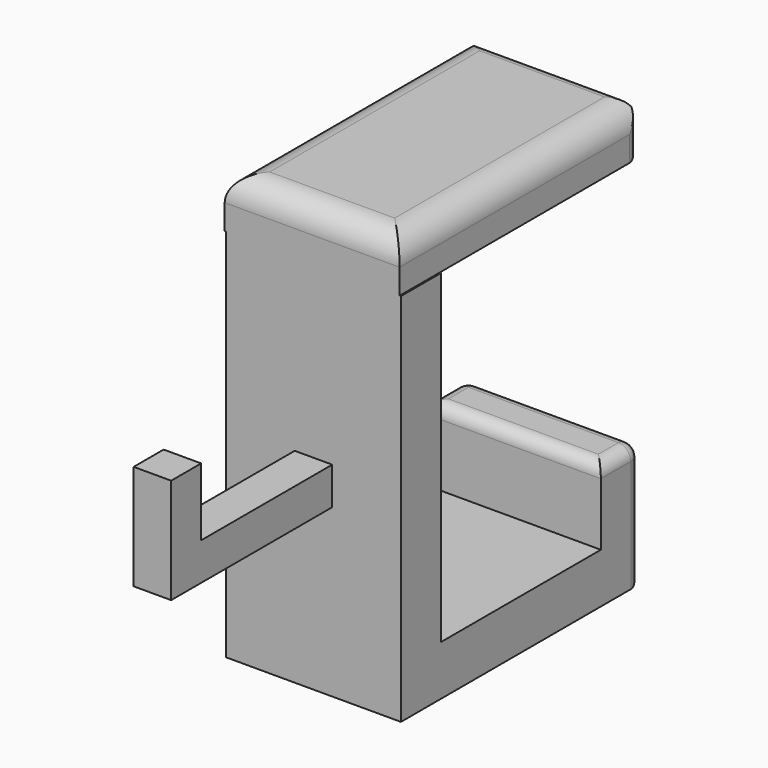
from build123d import *

# Parameters (mm, degrees)
F1_W         = 17.78
F1_H         = 30.48
F2_DEPTH     = 5.08
F3_W         = 17.78
F3_H         = 5.08
F4_DEPTH     = 38.1
F6_W         = 17.78
F6_H         = 5.08
F7_DEPTH     = 25.4
F9_W         = 17.78
F9_H         = 5.08
F10_DEPTH    = 7.62
F11_R        = 1.27
F12_R        = 1.27
F13_T1_DEPTH = 41.91
F13_T3_DEPTH = 30.48
F16_DEPTH    = 1.905


# Not quite as in the source:
# - a fillet or chamfer that OpenCascade refuses, or shapes differently, is made with other operations: its cross-section is extruded or revolved along the edge and cut away or added


with BuildPart() as f2:
    # F1 (on offset) → F2 (new body)
    with BuildSketch(Plane.XY.offset(25.4)):
        with Locations((-1.3240431021, 15.24)):
            Rectangle(F1_W, F1_H)
    extrude(amount=F2_DEPTH)

    # F3 (on offset) → F4 (join)
    with BuildSketch(Plane.XY.offset(25.4)):
        with Locations((-1.1914440245, 2.54)):
            Rectangle(F3_W, F3_H)
    extrude(amount=-F4_DEPTH)

    # F6 (on offset) → F7 (join)
    with BuildSketch(Plane(origin=(0, 5.08, 0), x_dir=(-1, 0, 0), z_dir=(0, 1, 0))):
        with Locations((1.1914440245, -10.16)):
            Rectangle(F6_W, F6_H)
    extrude(amount=F7_DEPTH)

    # F9 (on offset) → F10 (join)
    with BuildSketch(Plane.XY.offset(-7.62)):
        with Locations((-1.1914440245, 27.94)):
            Rectangle(F9_W, F9_H)
    extrude(amount=F10_DEPTH)

    # F11
    f11_edges = [f2.edges().sort_by_distance(p)[0] for p in [
        (-1.191444, 30.48, 0),
        (-10.081444, 27.94, 0),
        (-1.191444, 25.4, 0),
        (7.698556, 27.94, 0),
        (-1.191444, 30.48, -12.7),
        (-10.081444, 30.48, -6.35),
        (7.698556, 30.48, -6.35),
    ]]
    fillet(f11_edges, radius=F11_R)

    # F12
    f12_edges = [f2.edges().sort_by_distance(p)[0] for p in [
        (7.565957, 30.48, 27.94),
        (-10.214043, 30.48, 27.94),
        (-1.324043, 30.48, 25.4),
        (-1.324043, 30.48, 30.48),
    ]]
    fillet(f12_edges, radius=F12_R)

    # F13: fillet of radius 2.54 on 4 edges, made by hand

    # F13_s2 → F13_t1 (cut)
    with BuildSketch(Plane.XZ.offset(-35.56)):
        with BuildLine():
            ThreePointArc((-10.2140431021, 27.94), (-9.4700943263, 29.7360512242), (-7.6740431021, 30.48))
            Line((-7.6740431021, 30.48), (-10.2140431021, 30.48))
            Line((-10.2140431021, 30.48), (-10.2140431021, 27.94))
        make_face()
        with BuildLine():
            ThreePointArc((7.5659568979, 27.94), (6.8220081221, 29.7360512242), (5.0259568979, 30.48))
            Line((5.0259568979, 30.48), (7.5659568979, 30.48))
            Line((7.5659568979, 30.48), (7.5659568979, 27.94))
        make_face()
    extrude(amount=F13_T1_DEPTH, mode=Mode.SUBTRACT)

    # F13_s4 → F13_t3 (cut)
    with BuildSketch(Plane.YZ.offset(-16.5640431021)):
        with BuildLine():
            ThreePointArc((0, 27.94), (0.7439487758, 29.7360512242), (2.54, 30.48))
            Line((2.54, 30.48), (0, 30.48))
            Line((0, 30.48), (0, 27.94))
        make_face()
    extrude(amount=F13_T3_DEPTH, mode=Mode.SUBTRACT)

    # F15 (on offset) → F16 (join, symmetric)
    with BuildSketch(Plane.YZ.offset(-1.1914440245)):
        Polygon((-20.4633865505, 4.2401612736), (0, 4.2401612736), (0, 8.0501612736), (-16.6533865505, 8.0501612736), (-16.6533865505, 14.932741411), (-20.4633865505, 14.932741411), align=None)
    extrude(amount=F16_DEPTH, both=True)


solid = f2.part
